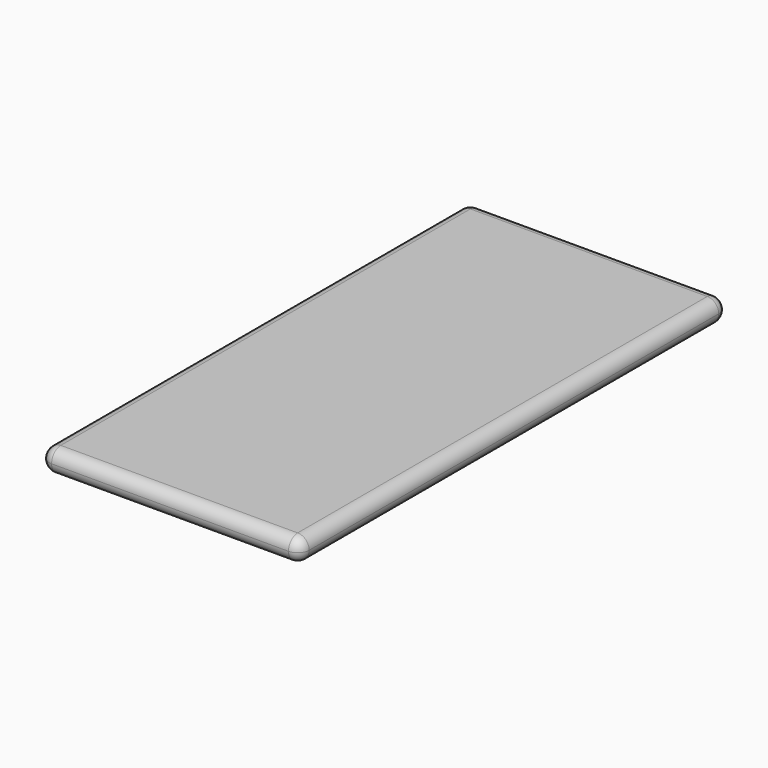
from build123d import *

# Parameters (mm, degrees)
F0_W     = 70.8
F0_H     = 145.75
F1_DEPTH = 6.26
F2_R     = 3.12999


# Not quite as in the source:
# - a fillet or chamfer is up to 0.001 mm smaller than in the source, because OpenCascade refuses the exact size


with BuildPart() as f1:
    # F0 (on Top) → F1 (new body)
    with BuildSketch(Plane.XY):
        Rectangle(F0_W, F0_H)
        with BuildLine():
            Line((-34.9, -69.245), (-34.9, 69.245))
            ThreePointArc((-34.9, 69.245), (-33.9832442251, 71.4582442251), (-31.77, 72.375))
            Line((-31.77, 72.375), (31.77, 72.375))
            ThreePointArc((31.77, 72.375), (33.9832442251, 71.4582442251), (34.9, 69.245))
            Line((34.9, 69.245), (34.9, -69.245))
            ThreePointArc((34.9, -69.245), (33.9832442251, -71.4582442251), (31.77, -72.375))
            Line((31.77, -72.375), (-31.77, -72.375))
            ThreePointArc((-31.77, -72.375), (-33.9832442251, -71.4582442251), (-34.9, -69.245))
        make_face(mode=Mode.SUBTRACT)
        with BuildLine():
            ThreePointArc((-31.77, 72.375), (-33.9832442251, 71.4582442251), (-34.9, 69.245))
            Line((-34.9, 69.245), (-34.9, -69.245))
            ThreePointArc((-34.9, -69.245), (-33.9832442251, -71.4582442251), (-31.77, -72.375))
            Line((-31.77, -72.375), (31.77, -72.375))
            ThreePointArc((31.77, -72.375), (33.9832442251, -71.4582442251), (34.9, -69.245))
            Line((34.9, -69.245), (34.9, 69.245))
            ThreePointArc((34.9, 69.245), (33.9832442251, 71.4582442251), (31.77, 72.375))
            Line((31.77, 72.375), (-31.77, 72.375))
        make_face()
    extrude(amount=-F1_DEPTH)

    # F2 (radius 3.13 in the source; OpenCascade refuses exactly that, so slightly less here)
    f2_edges = [f1.edges().sort_by_distance(p)[0] for p in [
        (35.4, 0, 0),
        (0, 72.875, 0),
        (-35.4, 0, 0),
        (0, -72.875, 0),
        (35.4, 0, -6.26),
        (0, 72.875, -6.26),
        (-35.4, 0, -6.26),
        (0, -72.875, -6.26),
        (35.4, -72.875, -3.13),
        (-35.4, -72.875, -3.13),
        (-35.4, 72.875, -3.13),
        (35.4, 72.875, -3.13),
    ]]
    fillet(f2_edges, radius=F2_R)


solid = f1.part
